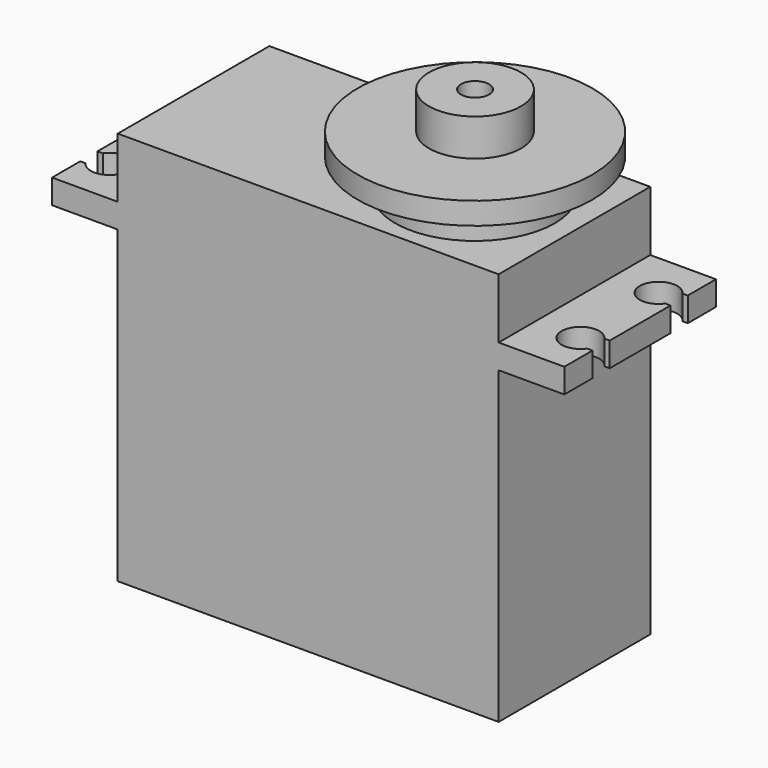
from build123d import *

# Parameters (mm, degrees)
F0_W          = 40.6
F0_H          = 20.2
F0_R          = 8.5
F0_R_2        = 2.95
F1_DEPTH      = 33
F1_DEPTH_BACK = 9
F2_DEPTH      = 2.6
F3_DEPTH      = 11.5
F4_DEPTH      = 15.8
F5_R          = 4.9
F5_R_2        = 2.95
F6_DEPTH      = 3.3
F6_DEPTH_BACK = 3
F7_START      = -0.95
F5_R_3        = 12.5
F7_DEPTH      = 2.35
F5_R_4        = 1.5
F8_DEPTH      = 3


# Not quite as in the source:
# - a feature names something its author has since deleted; it is built from what else it names


with BuildPart() as f1:
    # F0 (on Top) → F1 (new body, two sides)
    with BuildSketch(Plane.XY) as f1_sk:
        with Locations((-9.7, 0)):
            Rectangle(F0_W, F0_H)
        Circle(F0_R, mode=Mode.SUBTRACT)
        Circle(F0_R)
        Circle(F0_R_2, mode=Mode.SUBTRACT)
        Circle(F0_R_2)
    extrude(amount=-F1_DEPTH)
    extrude(f1_sk.sketch, amount=F1_DEPTH_BACK)

    # F0 (on Top) → F2 (join)
    with BuildSketch(Plane.XY):
        with BuildLine():
            Line((-30, -10.1), (-30, 10.1))
            Line((-30, 10.1), (-37, 10.1))
            Line((-37, 10.1), (-37, 6.35))
            Line((-37, 6.35), (-36.4363068172, 6.35))
            ThreePointArc((-36.4363068172, 6.35), (-32.8, 5.2), (-36.4363068172, 4.05))
            Line((-36.4363068172, 4.05), (-37, 4.05))
            Line((-37, 4.05), (-37, -4.05))
            Line((-37, -4.05), (-36.4363068172, -4.05))
            ThreePointArc((-36.4363068172, -4.05), (-32.8, -5.2), (-36.4363068172, -6.35))
            Line((-36.4363068172, -6.35), (-37, -6.35))
            Line((-37, -6.35), (-37, -10.1))
            Line((-37, -10.1), (-30, -10.1))
        make_face()
        with BuildLine():
            Line((17.6, 10.1), (10.6, 10.1))
            Line((10.6, 10.1), (10.6, -10.1))
            Line((10.6, -10.1), (17.6, -10.1))
            Line((17.6, -10.1), (17.6, -6.35))
            Line((17.6, -6.35), (17.0363068172, -6.35))
            ThreePointArc((17.0363068172, -6.35), (13.4, -5.2), (17.0363068172, -4.05))
            Line((17.0363068172, -4.05), (17.6, -4.05))
            Line((17.6, -4.05), (17.6, 4.05))
            Line((17.6, 4.05), (17.0363068172, 4.05))
            ThreePointArc((17.0363068172, 4.05), (13.4, 5.2), (17.0363068172, 6.35))
            Line((17.0363068172, 6.35), (17.6, 6.35))
            Line((17.6, 6.35), (17.6, 10.1))
        make_face()
    extrude(amount=F2_DEPTH)

    # F0 (on Top) → F3 (join)
    with BuildSketch(Plane.XY):
        Circle(F0_R)
        Circle(F0_R_2, mode=Mode.SUBTRACT)
        Circle(F0_R_2)
    extrude(amount=F3_DEPTH)

    # F0 (on Top) → F4 (join)
    with BuildSketch(Plane.XY):
        Circle(F0_R_2)
    extrude(amount=F4_DEPTH)


with BuildPart() as f6:
    # F5 (on face) → F6 (new body, two sides)
    with BuildSketch(Plane.XY.offset(15.8)) as f6_sk:
        Circle(F5_R)
        Circle(F5_R_2, mode=Mode.SUBTRACT)
    extrude(amount=-F6_DEPTH)
    extrude(f6_sk.sketch, amount=F6_DEPTH_BACK)

    # F5 (on face) → F7 (join)
    with BuildSketch(Plane.XY.offset(15.8).offset(F7_START)):
        Circle(F5_R_3)
        Circle(F5_R, mode=Mode.SUBTRACT)
        Circle(F5_R)
        Circle(F5_R_2, mode=Mode.SUBTRACT)
    extrude(amount=-F7_DEPTH)

    # F5 (on face) → F8 (join)
    with BuildSketch(Plane.XY.offset(15.8)):
        Circle(F5_R_2)
        Circle(F5_R_4, mode=Mode.SUBTRACT)
    extrude(amount=F8_DEPTH)


solid = Compound([f1.part, f6.part])
